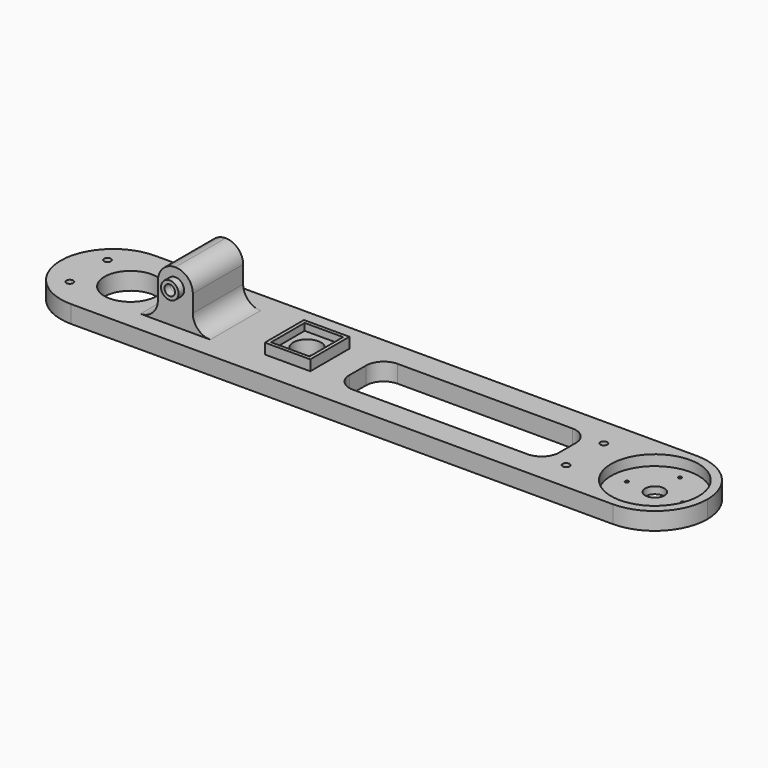
from build123d import *
from build123d import SkipClean  # not in build123d's __all__

# Parameters (mm, degrees)
F0_W      = 185
F0_H      = 30
F0_R      = 1
F0_W_2    = 60
F0_H_2    = 16
F1_DEPTH  = 5
F2_R      = 12.5
F2_R_2    = 0.5
F2_R_3    = 2.75
F3_DEPTH  = 3
F4_DEPTH  = 25
F5_R      = 14.99999
F2_R_4    = 7.5
F6_DEPTH  = 25
F2_W      = 10
F2_H      = 18
F7_DEPTH  = 15
F8_R      = 4.99999
F9_R      = 1.5
F10_DEPTH = 25
F9_R_2    = 2.5
F11_DEPTH = 2
F12_R     = 2.5
F12_R_2   = 1.5
F13_DEPTH = 2
F2_W_2    = 13
F2_H_2    = 14
F14_DEPTH = 3
F15_W     = 11
F15_H     = 12
F15_R     = 4
F16_DEPTH = 2
F17_DEPTH = 25
F18_R     = 5


# Not quite as in the source:
# - a fillet or chamfer is up to 0.001 mm smaller than in the source, because OpenCascade refuses the exact size
# - after a boolean that leaves OpenCascade's solid faulty, fix() repairs it


with BuildPart() as f1:
    # F0 (on Top) → F1 (new body)
    with BuildSketch(Plane.XY):
        with Locations((7.5, -11.8972941886)):
            Rectangle(F0_W, F0_H)
        with Locations((-77, -18.6472941886)):
            Circle(F0_R, mode=Mode.SUBTRACT)
        with Locations((30, -11.8972941886)):
            Rectangle(F0_W_2, F0_H_2, mode=Mode.SUBTRACT)
        with Locations((65, -18.6472941886)):
            Circle(F0_R, mode=Mode.SUBTRACT)
        with Locations((-77, -5.1472941886)):
            Circle(F0_R, mode=Mode.SUBTRACT)
        with Locations((65, -5.1472941886)):
            Circle(F0_R, mode=Mode.SUBTRACT)
    extrude(amount=F1_DEPTH)

    # F2 (on face) → F3 (cut)
    with BuildSketch(Plane.XY.offset(5)):
        with Locations((85, -11.8972941886)):
            Circle(F2_R)
        with Locations((85, -20.8972941886)):
            Circle(F2_R_2, mode=Mode.SUBTRACT)
        with Locations((85, -11.8972941886)):
            Circle(F2_R_3, mode=Mode.SUBTRACT)
        with Locations((77, -11.8972941886)):
            Circle(F2_R_2, mode=Mode.SUBTRACT)
        with Locations((93, -11.8972941886)):
            Circle(F2_R_2, mode=Mode.SUBTRACT)
        with Locations((85, -2.8972941886)):
            Circle(F2_R_2, mode=Mode.SUBTRACT)
    extrude(amount=-F3_DEPTH, mode=Mode.SUBTRACT)

    # F2 (on face) → F4 (cut)
    with BuildSketch(Plane.XY.offset(5)):
        with Locations((85, -11.8972941886)):
            Circle(F2_R_3)
        with Locations((85, -2.8972941886)):
            Circle(F2_R_2)
        with Locations((77, -11.8972941886)):
            Circle(F2_R_2)
        with Locations((85, -20.8972941886)):
            Circle(F2_R_2)
        with Locations((93, -11.8972941886)):
            Circle(F2_R_2)
    extrude(amount=-F4_DEPTH, mode=Mode.SUBTRACT)

    # F5 (radius 15 in the source; OpenCascade refuses exactly that, so slightly less here)
    f5_edges = [f1.edges().sort_by_distance(p)[0] for p in [
        (100, 3.102706, 2.5),
        (100, -26.897294, 2.5),
        (-85, -26.897294, 2.5),
        (-85, 3.102706, 2.5),
    ]]
    fillet(f5_edges, radius=F5_R)

    # F2 (on face) → F6 (cut)
    with BuildSketch(Plane.XY.offset(5)):
        with Locations((-65, -11.8972941886)):
            Circle(F2_R_4)
    extrude(amount=-F6_DEPTH, mode=Mode.SUBTRACT)

    # F2 (on face) → F7 (join)
    with BuildSketch(Plane.XY.offset(5)):
        with Locations((-45, -11.8972941886)):
            Rectangle(F2_W, F2_H)
    extrude(amount=F7_DEPTH)

    # F8 (radius 5 in the source; OpenCascade refuses exactly that, so slightly less here)
    f8_edges = [f1.edges().sort_by_distance(p)[0] for p in [
        (-50, -11.897294, 5),
        (-40, -11.897294, 20),
        (-50, -11.897294, 20),
        (-40, -11.897294, 5),
    ]]
    fillet(f8_edges, radius=F8_R)

    # F9 (on face) → F10 (cut)
    with BuildSketch(Plane.XZ.offset(20.8972941886)):
        with Locations((-45, 15)):
            Circle(F9_R)
    extrude(amount=-F10_DEPTH, mode=Mode.SUBTRACT)

    # F9 (on face) → F11 (join)
    with BuildSketch(Plane.XZ.offset(20.8972941886)):
        with Locations((-45, 15)):
            Circle(F9_R_2)
        with Locations((-45, 15)):
            Circle(F9_R, mode=Mode.SUBTRACT)
    extrude(amount=F11_DEPTH)

    # F12 (on face) → F13 (join)
    with BuildSketch(Plane(origin=(0, -2.8972941886, 0), x_dir=(-1, 0, 0), z_dir=(0, 1, 0))):
        with Locations((45, 15)):
            Circle(F12_R)
        with Locations((45, 15)):
            Circle(F12_R_2, mode=Mode.SUBTRACT)
    with SkipClean():  # cleaning this boolean's faces spoils the solid; the shape is the same uncleaned
        extrude(amount=F13_DEPTH)

    # F2 (on face) → F14 (join)
    with BuildSketch(Plane.XY.offset(5)):
        with Locations((-14.5, -11.8972941886)):
            Rectangle(F2_W_2, F2_H_2)
    extrude(amount=F14_DEPTH)

    add(f1.part.fix(), mode=Mode.REPLACE)

    # F15 (on face) → F16 (cut)
    with BuildSketch(Plane.XY.offset(8)):
        with Locations((-14.5, -11.8972941886)):
            Rectangle(F15_W, F15_H)
        with Locations((-14.5, -11.8972941886)):
            Circle(F15_R, mode=Mode.SUBTRACT)
    extrude(amount=-F16_DEPTH, mode=Mode.SUBTRACT)

    # F17 (cut): a face of the model
    f17_faces = [f1.faces().sort_by_distance(p)[0] for p in [
        (-14.5, -11.8972941886, 8),
    ]]
    extrude(f17_faces, amount=-F17_DEPTH, mode=Mode.SUBTRACT)

    # F18
    f18_edges = [f1.edges().sort_by_distance(p)[0] for p in [
        (0, -3.897294, 2.5),
        (0, -19.897294, 2.5),
        (60, -3.897294, 2.5),
        (60, -19.897294, 2.5),
    ]]
    fillet(f18_edges, radius=F18_R)


solid = f1.part
